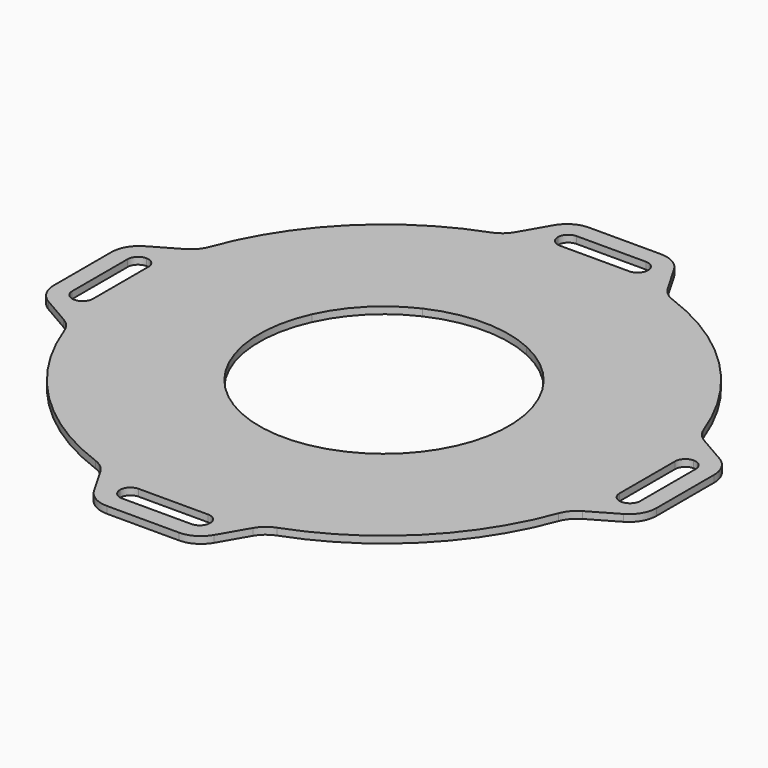
from build123d import *

# Parameters (mm, degrees)
F1_DEPTH        = 12.7
F2_DEPTH        = 25.4
F2_COPIES_COUNT = 4
F3_R            = 19.04999
F5_R            = 50.8


# Not quite as in the source:
# - a fillet or chamfer is up to 0.001 mm smaller than in the source, because OpenCascade refuses the exact size
# - a feature of the source that left no trace in its solid (it failed there, or was rolled back) is left out
# - a pattern or mirror of a feature is missing from the dataset's text; its kind, count and spacing are read off the source's solid


with BuildPart() as f1:
    # F0 (on Top) → F1 (new body)
    with BuildSketch(Plane.XY):
        with BuildLine():
            Line((552.45, 95.25), (473.1069620075, 95.25))
            ThreePointArc((473.1069620075, 95.25), (480.2208761939, 47.8609451179), (482.6, 0))
            ThreePointArc((482.6, 0), (480.2208761939, -47.8609451179), (473.1069620075, -95.25))
            Line((473.1069620075, -95.25), (552.45, -95.25))
            Line((552.45, -95.25), (552.45, 95.25))
        make_face()
        with BuildLine():
            Line((-207.8109657838, 95.25), (-473.1069620075, 95.25))
            ThreePointArc((-473.1069620075, 95.25), (-480.2208762804, 47.8609442495), (-482.6, -1.7456e-06))
            ThreePointArc((-482.6, -1.7456e-06), (-480.2208761073, -47.8609459864), (-473.1069620075, -95.25))
            Line((-473.1069620075, -95.25), (-207.8109657838, -95.25))
            ThreePointArc((-207.8109657838, -95.25), (-228.6, 0), (-207.8109657838, 95.25))
        make_face()
        with BuildLine():
            Line((473.1069620075, 95.25), (207.8109657838, 95.25))
            ThreePointArc((207.8109657838, 95.25), (223.3422785527, 48.7461445748), (228.6, 0))
            ThreePointArc((228.6, 0), (223.3422785527, -48.7461445748), (207.8109657838, -95.25))
            Line((207.8109657838, -95.25), (473.1069620075, -95.25))
            ThreePointArc((473.1069620075, -95.25), (480.2208761939, -47.8609451179), (482.6, 0))
            ThreePointArc((482.6, 0), (480.2208761939, 47.8609451179), (473.1069620075, 95.25))
        make_face()
        with BuildLine():
            ThreePointArc((-458.9465033909, 149.2342689375), (-466.8077665522, 122.4470052167), (-473.1069620075, 95.25))
            Line((-473.1069620075, 95.25), (-207.8109657838, 95.25))
            ThreePointArc((-207.8109657838, 95.25), (-161.6446101792, 161.6446101792), (-95.25, 207.8109657838))
            Line((-95.25, 207.8109657838), (-95.25, 473.1069620075))
            ThreePointArc((-95.25, 473.1069620075), (-122.4470052167, 466.8077665522), (-149.2342689375, 458.9465033909))
            ThreePointArc((-149.2342689375, 458.9465033909), (-341.2497326006, 341.2497326006), (-458.9465033909, 149.2342689375))
        make_face()
        with BuildLine():
            Line((-95.25, 473.1069620075), (-95.25, 207.8109657838))
            ThreePointArc((-95.25, 207.8109657838), (0, 228.6), (95.25, 207.8109657838))
            Line((95.25, 207.8109657838), (95.25, 473.1069620075))
            ThreePointArc((95.25, 473.1069620075), (0, 482.6), (-95.25, 473.1069620075))
        make_face()
        with BuildLine():
            Line((95.25, 473.1069620075), (95.25, 207.8109657838))
            ThreePointArc((95.25, 207.8109657838), (161.6446101792, 161.6446101792), (207.8109657838, 95.25))
            Line((207.8109657838, 95.25), (473.1069620075, 95.25))
            ThreePointArc((473.1069620075, 95.25), (466.8077665522, 122.4470052167), (458.9465033909, 149.2342689375))
            ThreePointArc((458.9465033909, 149.2342689375), (341.2497326006, 341.2497326006), (149.2342689375, 458.9465033909))
            ThreePointArc((149.2342689375, 458.9465033909), (122.4470052167, 466.8077665522), (95.25, 473.1069620075))
        make_face()
        with BuildLine():
            Line((-95.25, 552.45), (-95.25, 473.1069620075))
            ThreePointArc((-95.25, 473.1069620075), (0, 482.6), (95.25, 473.1069620075))
            Line((95.25, 473.1069620075), (95.25, 552.45))
            Line((95.25, 552.45), (-95.25, 552.45))
        make_face()
        with BuildLine():
            ThreePointArc((207.8109657838, -95.25), (161.6446101792, -161.6446101792), (95.25, -207.8109657838))
            Line((95.25, -207.8109657838), (95.25, -473.1069620075))
            ThreePointArc((95.25, -473.1069620075), (122.4470052167, -466.8077665522), (149.2342689375, -458.9465033909))
            ThreePointArc((149.2342689375, -458.9465033909), (341.2497326006, -341.2497326006), (458.9465033909, -149.2342689375))
            ThreePointArc((458.9465033909, -149.2342689375), (466.8077665522, -122.4470052167), (473.1069620075, -95.25))
            Line((473.1069620075, -95.25), (207.8109657838, -95.25))
        make_face()
        with BuildLine():
            ThreePointArc((95.25, -207.8109657838), (0, -228.6), (-95.25, -207.8109657838))
            Line((-95.25, -207.8109657838), (-95.25, -473.1069620075))
            ThreePointArc((-95.25, -473.1069620075), (0, -482.6), (95.25, -473.1069620075))
            Line((95.25, -473.1069620075), (95.25, -207.8109657838))
        make_face()
        with BuildLine():
            Line((-207.8109657838, -95.25), (-473.1069620075, -95.25))
            ThreePointArc((-473.1069620075, -95.25), (-466.8077665522, -122.4470052167), (-458.9465033909, -149.2342689375))
            ThreePointArc((-458.9465033909, -149.2342689375), (-341.2497326006, -341.2497326006), (-149.2342689375, -458.9465033909))
            ThreePointArc((-149.2342689375, -458.9465033909), (-122.4470052167, -466.8077665522), (-95.25, -473.1069620075))
            Line((-95.25, -473.1069620075), (-95.25, -207.8109657838))
            ThreePointArc((-95.25, -207.8109657838), (-161.6446101792, -161.6446101792), (-207.8109657838, -95.25))
        make_face()
        with BuildLine():
            ThreePointArc((95.25, -473.1069620075), (0, -482.6), (-95.25, -473.1069620075))
            Line((-95.25, -473.1069620075), (-95.25, -552.45))
            Line((-95.25, -552.45), (95.25, -552.45))
            Line((95.25, -552.45), (95.25, -473.1069620075))
        make_face()
        with BuildLine():
            Line((-473.1069620075, 95.25), (-552.45, 95.25))
            Line((-552.45, 95.25), (-552.45, -95.25))
            Line((-552.45, -95.25), (-473.1069620075, -95.25))
            ThreePointArc((-473.1069620075, -95.25), (-480.2208761073, -47.8609459864), (-482.6, -1.7456e-06))
            ThreePointArc((-482.6, -1.7456e-06), (-480.2208762804, 47.8609442495), (-473.1069620075, 95.25))
        make_face()
        Polygon((-482.6, 82.55), (-482.6, -1.7456e-06), (-482.6, -82.55), (-520.7, -82.55), (-520.7, 82.55), align=None, mode=Mode.SUBTRACT)
        Polygon((-482.6, -82.55), (-482.6, -1.7456e-06), (-482.6, 82.55), (-520.7, 82.55), (-520.7, -82.55), align=None)
        with BuildLine():
            Line((-458.9465033909, 149.2342689375), (-552.45, 95.25))
            Line((-552.45, 95.25), (-473.1069620075, 95.25))
            ThreePointArc((-473.1069620075, 95.25), (-466.8077665522, 122.4470052167), (-458.9465033909, 149.2342689375))
        make_face()
        with BuildLine():
            Line((-473.1069620075, -95.25), (-552.45, -95.25))
            Line((-552.45, -95.25), (-458.9465033909, -149.2342689375))
            ThreePointArc((-458.9465033909, -149.2342689375), (-466.8077665522, -122.4470052167), (-473.1069620075, -95.25))
        make_face()
        with BuildLine():
            Line((-95.25, 552.45), (-149.2342689375, 458.9465033909))
            ThreePointArc((-149.2342689375, 458.9465033909), (-122.4470052167, 466.8077665522), (-95.25, 473.1069620075))
            Line((-95.25, 473.1069620075), (-95.25, 552.45))
        make_face()
        with BuildLine():
            Line((95.25, 552.45), (95.25, 473.1069620075))
            ThreePointArc((95.25, 473.1069620075), (122.4470052167, 466.8077665522), (149.2342689375, 458.9465033909))
            Line((149.2342689375, 458.9465033909), (95.25, 552.45))
        make_face()
        with BuildLine():
            ThreePointArc((458.9465033909, 149.2342689375), (466.8077665522, 122.4470052167), (473.1069620075, 95.25))
            Line((473.1069620075, 95.25), (552.45, 95.25))
            Line((552.45, 95.25), (458.9465033909, 149.2342689375))
        make_face()
        with BuildLine():
            Line((552.45, -95.25), (473.1069620075, -95.25))
            ThreePointArc((473.1069620075, -95.25), (466.8077665522, -122.4470052167), (458.9465033909, -149.2342689375))
            Line((458.9465033909, -149.2342689375), (552.45, -95.25))
        make_face()
        with BuildLine():
            ThreePointArc((149.2342689375, -458.9465033909), (122.4470052167, -466.8077665522), (95.25, -473.1069620075))
            Line((95.25, -473.1069620075), (95.25, -552.45))
            Line((95.25, -552.45), (149.2342689375, -458.9465033909))
        make_face()
        with BuildLine():
            ThreePointArc((-95.25, -473.1069620075), (-122.4470052167, -466.8077665522), (-149.2342689375, -458.9465033909))
            Line((-149.2342689375, -458.9465033909), (-95.25, -552.45))
            Line((-95.25, -552.45), (-95.25, -473.1069620075))
        make_face()
    extrude(amount=-F1_DEPTH)

    # F0 (on Top) → F2 (cut)
    with BuildSketch(Plane.XY):
        Polygon((-482.6, -82.55), (-482.6, -1.7456e-06), (-482.6, 82.55), (-520.7, 82.55), (-520.7, -82.55), align=None)
    f2 = extrude(amount=-F2_DEPTH, mode=Mode.SUBTRACT)

    # F2_copies: F2 ×4 about axis
    f2_copies_axis = Axis((0, 0, 0), (0, 0, 1))
    for i in range(1, F2_COPIES_COUNT):
        add(f2.rotate(f2_copies_axis, i * 360 / F2_COPIES_COUNT), mode=Mode.SUBTRACT)

    # F3 (radius 19.05 in the source; OpenCascade refuses exactly that, so slightly less here)
    f3_edges = [f1.edges().sort_by_distance(p)[0] for p in [
        (-520.7, -82.55, -6.35),
        (-482.6, -82.55, -6.35),
        (-520.7, 82.55, -6.35),
        (-482.6, 82.55, -6.35),
        (-82.55, -520.7, -6.35),
        (-82.55, -482.6, -6.35),
        (82.55, -482.6, -6.35),
        (82.55, -520.7, -6.35),
        (520.7, -82.55, -6.35),
        (482.6, -82.55, -6.35),
        (482.6, 82.55, -6.35),
        (520.7, 82.55, -6.35),
        (82.55, 520.7, -6.35),
        (82.55, 482.6, -6.35),
        (-82.55, 520.7, -6.35),
        (-82.55, 482.6, -6.35),
    ]]
    fillet(f3_edges, radius=F3_R)

    # F5
    f5_edges = [f1.edges().sort_by_distance(p)[0] for p in [
        (-149.234269, -458.946503, -6.35),
        (-95.25, -552.45, -6.35),
        (95.25, -552.45, -6.35),
        (149.234269, -458.946503, -6.35),
        (458.946503, -149.234269, -6.35),
        (552.45, -95.25, -6.35),
        (552.45, 95.25, -6.35),
        (458.946503, 149.234269, -6.35),
        (149.234269, 458.946503, -6.35),
        (95.25, 552.45, -6.35),
        (-95.25, 552.45, -6.35),
        (-149.234269, 458.946503, -6.35),
        (-458.946503, 149.234269, -6.35),
        (-552.45, 95.25, -6.35),
        (-552.45, -95.25, -6.35),
        (-458.946503, -149.234269, -6.35),
    ]]
    fillet(f5_edges, radius=F5_R)


solid = f1.part
